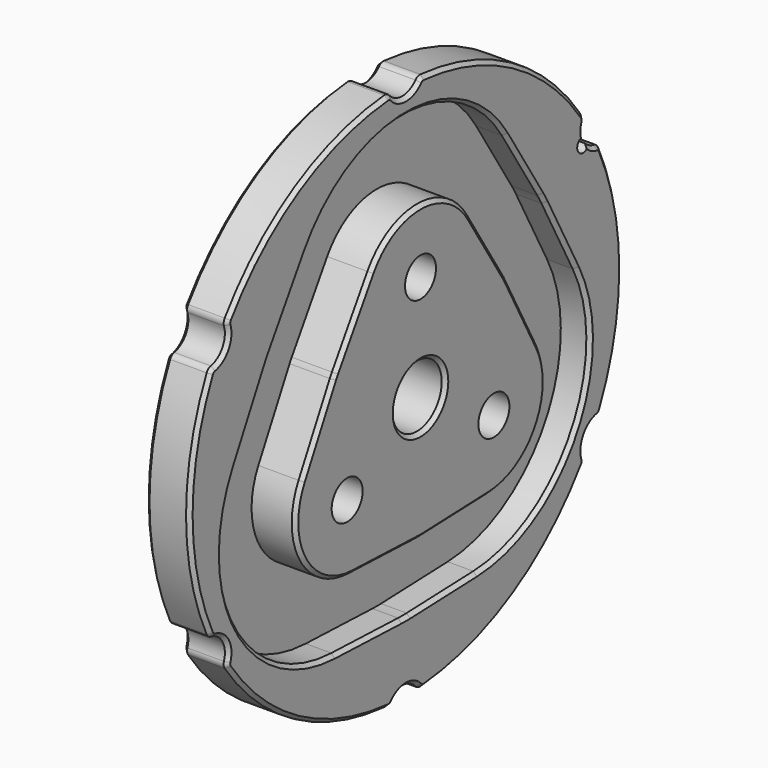
from build123d import *

# Parameters (mm, degrees)
F0_R     = 2.65
F0_R_2   = 4.25
F1_DEPTH = 6
F2_DEPTH = 4
F3_DEPTH = 2
F4_SIZE  = 0.5


with BuildPart() as f1:
    # F0 (on Right) → F1 (new body)
    with BuildSketch(Plane.YZ):
        with BuildLine():
            ThreePointArc((-2.2515407231, 36.53242851), (-2.6294191421, 36.8013801393), (-3.0879953604, 36.8709138028))
            ThreePointArc((-3.0879953604, 36.8709138028), (-18.5, 32.04293994), (-30.3871503338, 21.1097393303))
            ThreePointArc((-30.3871503338, 21.1097393303), (-30.5562205239, 20.6778338439), (-30.5122407901, 20.2161057189))
            ThreePointArc((-30.5122407901, 20.2161057189), (-30.7524645978, 17.7549437138), (-32.7637815132, 16.3163227911))
            ThreePointArc((-32.7637815132, 16.3163227911), (-33.185639666, 16.1235462954), (-33.4751456942, 15.7611744725))
            ThreePointArc((-33.4751456942, 15.7611744725), (-37, 0), (-33.4751456942, -15.7611744725))
            ThreePointArc((-33.4751456942, -15.7611744725), (-33.185639666, -16.1235462954), (-32.7637815132, -16.3163227911))
            ThreePointArc((-32.7637815132, -16.3163227911), (-30.7524645978, -17.7549437138), (-30.5122407901, -20.2161057189))
            ThreePointArc((-30.5122407901, -20.2161057189), (-30.5562205239, -20.6778338439), (-30.3871503338, -21.1097393303))
            ThreePointArc((-30.3871503338, -21.1097393303), (-18.5, -32.04293994), (-3.0879953604, -36.8709138028))
            ThreePointArc((-3.0879953604, -36.8709138028), (-2.6294191421, -36.8013801393), (-2.2515407231, -36.53242851))
            ThreePointArc((-2.2515407231, -36.53242851), (0, -35.5098874275), (2.2515407231, -36.53242851))
            ThreePointArc((2.2515407231, -36.53242851), (2.6294191421, -36.8013801393), (3.0879953604, -36.8709138028))
            ThreePointArc((3.0879953604, -36.8709138028), (18.5, -32.04293994), (30.3871503338, -21.1097393303))
            ThreePointArc((30.3871503338, -21.1097393303), (30.5562205239, -20.6778338439), (30.5122407901, -20.2161057189))
            ThreePointArc((30.5122407901, -20.2161057189), (30.7524645978, -17.7549437138), (32.7637815132, -16.3163227911))
            ThreePointArc((32.7637815132, -16.3163227911), (33.185639666, -16.1235462954), (33.4751456942, -15.7611744725))
            ThreePointArc((33.4751456942, -15.7611744725), (37, 0), (33.4751456942, 15.7611744725))
            ThreePointArc((33.4751456942, 15.7611744725), (33.185639666, 16.1235462954), (32.7637815132, 16.3163227911))
            ThreePointArc((32.7637815132, 16.3163227911), (31.941237039, 16.6082774884), (31.2380455813, 17.1253255822))
            ThreePointArc((31.2380455813, 17.1253255822), (29.4448637287, 17), (30.449989793, 18.4902782469))
            ThreePointArc((30.449989793, 18.4902782469), (30.3538087376, 19.3577839598), (30.5122407901, 20.2161057189))
            ThreePointArc((30.5122407901, 20.2161057189), (30.5562205239, 20.6778338439), (30.3871503338, 21.1097393303))
            ThreePointArc((30.3871503338, 21.1097393303), (18.5, 32.04293994), (3.0879953604, 36.8709138028))
            ThreePointArc((3.0879953604, 36.8709138028), (2.6294191421, 36.8013801393), (2.2515407231, 36.53242851))
            ThreePointArc((2.2515407231, 36.53242851), (0, 35.5098874275), (-2.2515407231, 36.53242851))
        make_face()
        with BuildLine():
            Line((-23.0952370323, 14.180454946), (-17.0328632471, 23.8484731203))
            ThreePointArc((-17.0328632471, 23.8484731203), (0.0002590164, 33.2703478915), (17.0295377344, 23.8415279974))
            Line((17.0295377344, 23.8415279974), (23.0899184639, 14.167925942))
            ThreePointArc((23.0899184639, 14.167925942), (23.4636524397, 13.5467460522), (23.8147430167, 12.9124929901))
            Line((23.8147430167, 12.9124929901), (29.162137778, 2.827248294))
            ThreePointArc((29.162137778, 2.827248294), (28.813095975, -16.6349496309), (12.1369519401, -26.6751288313))
            Line((12.1369519401, -26.6751288313), (0.7330157043, -27.0912894495))
            ThreePointArc((0.7330157043, -27.0912894495), (0, -27.1046598669), (-0.7330157043, -27.0912894495))
            Line((-0.7330157043, -27.0912894495), (-12.1441739659, -26.6748652799))
            ThreePointArc((-12.1441739659, -26.6748652799), (-28.8182692269, -16.6382354957), (-29.1731979579, 2.8202694775))
            Line((-29.1731979579, 2.8202694775), (-23.8282527367, 12.9108345034))
            ThreePointArc((-23.8282527367, 12.9108345034), (-23.4733240056, 13.5523299334), (-23.0952370323, 14.180454946))
        make_face(mode=Mode.SUBTRACT)
        with BuildLine():
            ThreePointArc((17.0295377344, 23.8415279974), (0.0002590164, 33.2703478915), (-17.0328632471, 23.8484731203))
            Line((-17.0328632471, 23.8484731203), (-23.0952370323, 14.180454946))
            ThreePointArc((-23.0952370323, 14.180454946), (-23.4733240056, 13.5523299334), (-23.8282527367, 12.9108345034))
            Line((-23.8282527367, 12.9108345034), (-29.1731979579, 2.8202694775))
            ThreePointArc((-29.1731979579, 2.8202694775), (-28.8182692269, -16.6382354957), (-12.1441739659, -26.6748652799))
            Line((-12.1441739659, -26.6748652799), (-0.7330157043, -27.0912894495))
            ThreePointArc((-0.7330157043, -27.0912894495), (0, -27.1046598669), (0.7330157043, -27.0912894495))
            Line((0.7330157043, -27.0912894495), (12.1369519401, -26.6751288313))
            ThreePointArc((12.1369519401, -26.6751288313), (28.813095975, -16.6349496309), (29.162137778, 2.827248294))
            Line((29.162137778, 2.827248294), (23.8147430167, 12.9124929901))
            ThreePointArc((23.8147430167, 12.9124929901), (23.4636524397, 13.5467460522), (23.0899184639, 14.167925942))
            Line((23.0899184639, 14.167925942), (17.0295377344, 23.8415279974))
        make_face()
        with BuildLine():
            Line((-14.5383641102, 8.8148297318), (-8.4759903249, 18.482847906))
            ThreePointArc((-8.4759903249, 18.482847906), (-0.0018003141, 23.1703476982), (8.4704774851, 18.4793926211))
            Line((8.4704774851, 18.4793926211), (14.5308582146, 8.8057905657))
            ThreePointArc((14.5308582146, 8.8057905657), (14.7167955123, 8.4967458506), (14.8914674376, 8.1811970698))
            Line((14.8914674376, 8.1811970698), (20.2388621989, -1.9040476263))
            ThreePointArc((20.2388621989, -1.9040476263), (20.0652095641, -11.5867329668), (11.7686206585, -16.5818468966))
            Line((11.7686206585, -16.5818468966), (0.3646844227, -16.9980075148))
            ThreePointArc((0.3646844227, -16.9980075148), (0, -17.0046594636), (-0.3646844227, -16.9980075148))
            Line((-0.3646844227, -16.9980075148), (-11.7758426843, -16.5815833453))
            ThreePointArc((-11.7758426843, -16.5815833453), (-20.0714122995, -11.5882352941), (-20.2479937541, -1.9073872429))
            Line((-20.2479937541, -1.9073872429), (-14.9030485329, 8.183177783))
            ThreePointArc((-14.9030485329, 8.183177783), (-14.7264670782, 8.5023297318), (-14.5383641102, 8.8148297318))
        make_face(mode=Mode.SUBTRACT)
        with BuildLine():
            ThreePointArc((8.4704774851, 18.4793926211), (-0.0018003141, 23.1703476982), (-8.4759903249, 18.482847906))
            Line((-8.4759903249, 18.482847906), (-14.5383641102, 8.8148297318))
            ThreePointArc((-14.5383641102, 8.8148297318), (-14.7264670782, 8.5023297318), (-14.9030485329, 8.183177783))
            Line((-14.9030485329, 8.183177783), (-20.2479937541, -1.9073872429))
            ThreePointArc((-20.2479937541, -1.9073872429), (-20.0714122995, -11.5882352941), (-11.7758426843, -16.5815833453))
            Line((-11.7758426843, -16.5815833453), (-0.3646844227, -16.9980075148))
            ThreePointArc((-0.3646844227, -16.9980075148), (0, -17.0046594636), (0.3646844227, -16.9980075148))
            Line((0.3646844227, -16.9980075148), (11.7686206585, -16.5818468966))
            ThreePointArc((11.7686206585, -16.5818468966), (20.0652095641, -11.5867329668), (20.2388621989, -1.9040476263))
            Line((20.2388621989, -1.9040476263), (14.8914674376, 8.1811970698))
            ThreePointArc((14.8914674376, 8.1811970698), (14.7167955123, 8.4967458506), (14.5308582146, 8.8057905657))
            Line((14.5308582146, 8.8057905657), (8.4704774851, 18.4793926211))
        make_face()
        with Locations((-12.5573683549, -7.25)):
            Circle(F0_R, mode=Mode.SUBTRACT)
        with Locations((12.5573683549, -7.25)):
            Circle(F0_R, mode=Mode.SUBTRACT)
        Circle(F0_R_2, mode=Mode.SUBTRACT)
        with Locations((0, 14.5)):
            Circle(F0_R, mode=Mode.SUBTRACT)
    extrude(amount=-F1_DEPTH)

    # F0 (on Right) → F2 (cut)
    with BuildSketch(Plane.YZ):
        with BuildLine():
            ThreePointArc((17.0295377344, 23.8415279974), (0.0002590164, 33.2703478915), (-17.0328632471, 23.8484731203))
            Line((-17.0328632471, 23.8484731203), (-23.0952370323, 14.180454946))
            ThreePointArc((-23.0952370323, 14.180454946), (-23.4733240056, 13.5523299334), (-23.8282527367, 12.9108345034))
            Line((-23.8282527367, 12.9108345034), (-29.1731979579, 2.8202694775))
            ThreePointArc((-29.1731979579, 2.8202694775), (-28.8182692269, -16.6382354957), (-12.1441739659, -26.6748652799))
            Line((-12.1441739659, -26.6748652799), (-0.7330157043, -27.0912894495))
            ThreePointArc((-0.7330157043, -27.0912894495), (0, -27.1046598669), (0.7330157043, -27.0912894495))
            Line((0.7330157043, -27.0912894495), (12.1369519401, -26.6751288313))
            ThreePointArc((12.1369519401, -26.6751288313), (28.813095975, -16.6349496309), (29.162137778, 2.827248294))
            Line((29.162137778, 2.827248294), (23.8147430167, 12.9124929901))
            ThreePointArc((23.8147430167, 12.9124929901), (23.4636524397, 13.5467460522), (23.0899184639, 14.167925942))
            Line((23.0899184639, 14.167925942), (17.0295377344, 23.8415279974))
        make_face()
        with BuildLine():
            Line((-14.5383641102, 8.8148297318), (-8.4759903249, 18.482847906))
            ThreePointArc((-8.4759903249, 18.482847906), (-0.0018003141, 23.1703476982), (8.4704774851, 18.4793926211))
            Line((8.4704774851, 18.4793926211), (14.5308582146, 8.8057905657))
            ThreePointArc((14.5308582146, 8.8057905657), (14.7167955123, 8.4967458506), (14.8914674376, 8.1811970698))
            Line((14.8914674376, 8.1811970698), (20.2388621989, -1.9040476263))
            ThreePointArc((20.2388621989, -1.9040476263), (20.0652095641, -11.5867329668), (11.7686206585, -16.5818468966))
            Line((11.7686206585, -16.5818468966), (0.3646844227, -16.9980075148))
            ThreePointArc((0.3646844227, -16.9980075148), (0, -17.0046594636), (-0.3646844227, -16.9980075148))
            Line((-0.3646844227, -16.9980075148), (-11.7758426843, -16.5815833453))
            ThreePointArc((-11.7758426843, -16.5815833453), (-20.0714122995, -11.5882352941), (-20.2479937541, -1.9073872429))
            Line((-20.2479937541, -1.9073872429), (-14.9030485329, 8.183177783))
            ThreePointArc((-14.9030485329, 8.183177783), (-14.7264670782, 8.5023297318), (-14.5383641102, 8.8148297318))
        make_face(mode=Mode.SUBTRACT)
    extrude(amount=-F2_DEPTH, mode=Mode.SUBTRACT)

    # F3 (add): a face of the model
    f3_faces = [f1.faces().sort_by_distance(p)[0] for p in [
        (0, -11.0097556238, 13.3369283968),
    ]]
    extrude(f3_faces, amount=F3_DEPTH)

    # F4
    f4_edges = [f1.edges().sort_by_distance(p)[0] for p in [
        (-6, 18.5, -32.04294),
        (0, 18.5, -32.04294),
        (0, 28.813096, -16.63495),
        (2, 20.06521, -11.586733),
        (2, -4.25, 0),
        (0, 30.556221, 20.677834),
        (-6, 30.556221, 20.677834),
        (0, 30.353809, 19.357784),
        (-6, 30.353809, 19.357784),
        (0, 18.5, 32.04294),
        (-6, 18.5, 32.04294),
        (0, 2.629419, 36.80138),
        (0, 31.941237, 16.608277),
        (0, 0, 35.509887),
        (0, 33.18564, 16.123546),
        (0, -2.629419, 36.80138),
        (0, 37, 0),
        (0, -18.5, 32.04294),
        (0, 33.18564, -16.123546),
        (0, -30.556221, 20.677834),
        (0, 30.752465, -17.754944),
        (0, -30.752465, 17.754944),
        (0, 30.556221, -20.677834),
        (0, -33.18564, 16.123546),
        (0, -37, 0),
        (0, 2.629419, -36.80138),
        (0, -33.18564, -16.123546),
        (0, 0, -35.509887),
        (0, -30.752465, -17.754944),
        (0, -2.629419, -36.80138),
        (0, -30.556221, -20.677834),
        (0, -18.5, -32.04294),
        (0, 23.463652, 13.546746),
        (0, 20.059728, 19.004727),
        (0, 0.000259, 33.270348),
        (0, -20.06405, 19.014464),
        (0, -23.473324, 13.55233),
        (0, -26.500725, 7.865552),
        (0, -28.818269, -16.638235),
        (0, -6.438595, -26.883077),
        (0, 0, -27.10466),
        (0, 6.434984, -26.883209),
        (0, 26.48844, 7.869871),
        (-6, 2.629419, 36.80138),
        (-6, 0, 35.509887),
        (-6, -2.629419, 36.80138),
        (-6, -18.5, 32.04294),
        (-6, -30.556221, 20.677834),
        (-6, -30.752465, 17.754944),
        (-6, -33.18564, 16.123546),
        (-6, -37, 0),
        (-6, -33.18564, -16.123546),
        (-6, -30.752465, -17.754944),
        (-6, -30.556221, -20.677834),
        (-6, -18.5, -32.04294),
        (-6, -2.629419, -36.80138),
        (-6, 0, -35.509887),
        (-6, 2.629419, -36.80138),
        (-6, 30.556221, -20.677834),
        (-6, 30.752465, -17.754944),
        (-6, 33.18564, -16.123546),
        (-6, 37, 0),
        (-6, 33.18564, 16.123546),
        (-6, 31.941237, 16.608277),
        (2, -11.507177, 13.648839),
        (2, -0.0018, 23.170348),
        (2, 11.500668, 13.642592),
        (2, 14.716796, 8.496746),
        (2, 17.565165, 3.138575),
        (2, 6.066653, -16.789927),
        (2, 0, -17.004659),
        (2, -6.070264, -16.789795),
        (2, -20.071412, -11.588235),
        (2, -17.575521, 3.137895),
        (2, -14.726467, 8.50233),
    ]]
    chamfer(f4_edges, length=F4_SIZE)


solid = f1.part
